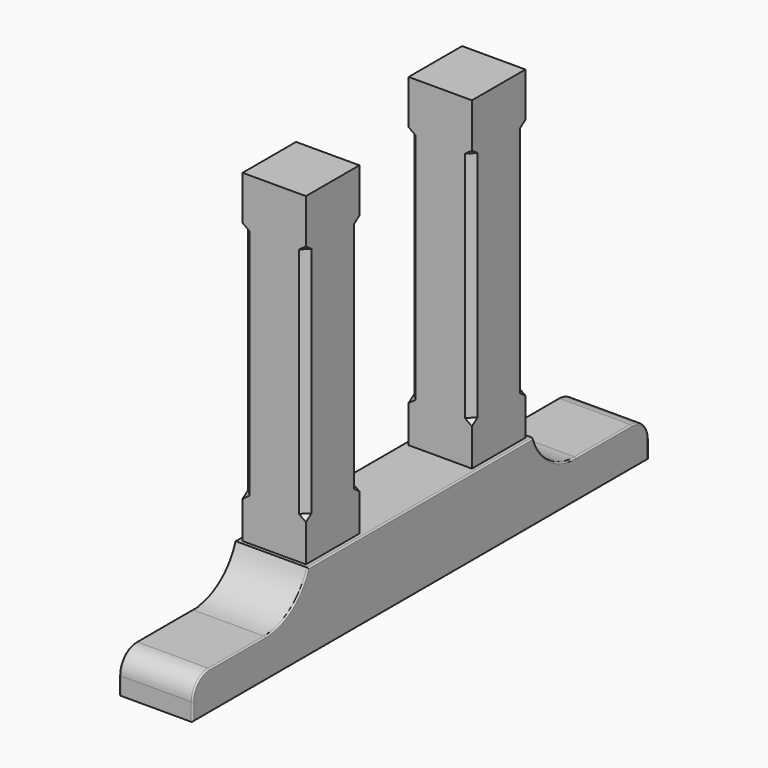
from build123d import *

# Parameters (mm, degrees)
F1_DEPTH      = 52
F1_DEPTH_BACK = 52
F0_W          = 95
F0_H          = 460.873763546
F2_DEPTH      = 45
F2_DEPTH_BACK = 45
F3_R          = 30
F4_T1_DEPTH   = 104
F5_T1_DEPTH   = 104
F6_SIZE       = 10
F7_W          = 90
F7_H          = 95
F8_DEPTH      = 50
F9_W          = 90
F9_H          = 95
F10_DEPTH     = 60
F11_T4_DEPTH  = 65.575795383
F11_T10_DEPTH = 65.575795383
F11_T16_DEPTH = 65.575795383
F11_T22_DEPTH = 65.575795383
F11_T28_DEPTH = 65.575795383
F11_T34_DEPTH = 65.575795383
F11_T40_DEPTH = 65.575795383
F11_T46_DEPTH = 65.575795383
F12_T4_DEPTH  = 65.575795383
F12_T10_DEPTH = 65.575795383
F12_T16_DEPTH = 65.575795383
F12_T22_DEPTH = 65.575795383
F12_T28_DEPTH = 65.575795383
F12_T34_DEPTH = 65.575795383
F12_T40_DEPTH = 65.575795383
F12_T46_DEPTH = 65.575795383
F13_R         = 2


# Not quite as in the source:
# - a fillet or chamfer that OpenCascade refuses, or shapes differently, is made with other operations: its cross-section is extruded or revolved along the edge and cut away or added


with BuildPart() as f1:
    # F0 (on Right) → F1 (new body, two sides)
    with BuildSketch(Plane.YZ) as f1_sk:
        Polygon((-405, 55), (-405, 0), (405, 0), (405, 55), (200, 55), (200, 110), (195, 110), (100, 110), (0, 110), (-100, 110), (-195, 110), (-200, 110), (-200, 55), align=None)
    extrude(amount=F1_DEPTH)
    extrude(f1_sk.sketch, amount=-F1_DEPTH_BACK)

    # F0 (on Right) → F2 (join, two sides)
    with BuildSketch(Plane.YZ) as f2_sk:
        with Locations((-147.5, 340.436881773)):
            Rectangle(F0_W, F0_H)
        with Locations((147.5, 340.436881773)):
            Rectangle(F0_W, F0_H)
    extrude(amount=-F2_DEPTH)
    extrude(f2_sk.sketch, amount=F2_DEPTH_BACK)

    # F3
    f3_edges = [f1.edges().sort_by_distance(p)[0] for p in [
        (0, 405, 55),
        (0, -405, 55),
    ]]
    fillet(f3_edges, radius=F3_R)

    # F4: fillet of radius 80 on 1 edges, made by hand

    # F4_s2 → F4_t1 (join)
    with BuildSketch(Plane.YZ.offset(-52)):
        with BuildLine():
            ThreePointArc((275.9934207679, 55), (229.0892631696, 70.1925930159), (200, 110))
            Line((200, 110), (200, 55))
            Line((200, 55), (275.9934207679, 55))
        make_face()
    extrude(amount=F4_T1_DEPTH)

    # F5: fillet of radius 80 on 1 edges, made by hand

    # F5_s2 → F5_t1 (join)
    with BuildSketch(Plane.YZ.offset(-52)):
        with BuildLine():
            ThreePointArc((-275.9934207679, 55), (-229.0892631696, 70.1925930159), (-200, 110))
            Line((-200, 110), (-200, 55))
            Line((-200, 55), (-275.9934207679, 55))
        make_face()
    extrude(amount=F5_T1_DEPTH)

    # F6
    f6_edges = [f1.edges().sort_by_distance(p)[0] for p in [
        (45, -195, 340.436882),
        (45, -100, 340.436882),
        (45, 100, 340.436882),
        (-45, -195, 340.436882),
        (-45, -100, 340.436882),
        (-45, 100, 340.436882),
        (-45, 195, 340.436882),
        (45, 195, 340.436882),
    ]]
    chamfer(f6_edges, length=F6_SIZE)

    # F7 (on face) → F8 (join)
    with BuildSketch(Plane.XY.offset(110)):
        with Locations((0, -147.5)):
            Rectangle(F7_W, F7_H)
        with Locations((0, 147.5)):
            Rectangle(F7_W, F7_H)
    extrude(amount=F8_DEPTH)

    # F9 (on face) → F10 (join)
    with BuildSketch(Plane.XY.offset(570.873763546)):
        Polygon((45, -110), (45, -100), (35, -100), align=None)
        Polygon((-45, -110), (-35, -100), (-45, -100), align=None)
        Polygon((45, -195), (45, -185), (35, -195), align=None)
        Polygon((-35, -195), (-45, -185), (-45, -195), align=None)
        with Locations((0, 147.5)):
            Rectangle(F9_W, F9_H)
        Polygon((45, -110), (35, -100), (-35, -100), (-45, -110), (-45, -185), (-35, -195), (35, -195), (45, -185), align=None)
    extrude(amount=-F10_DEPTH)

    # F11: chamfer of 10 on 8 edges, made by hand


with BuildPart() as f11_tool2:
    # F11_s3 → F11_t4 (new body)
    with BuildSketch(Plane(origin=(-98.1845447985, -98.1845447985, 0), x_dir=(0, 0, 1), z_dir=(0.7071067812, 0.7071067812, 0))):
        Polygon((510.873763546, 172.6345596729), (500.873763546, 162.6345596729), (510.873763546, 162.6345596729), align=None)
    extrude(amount=F11_T4_DEPTH)

    split(bisect_by=Plane.YZ.offset(45), keep=Keep.BOTTOM)

    split(bisect_by=Plane.XZ.offset(195), keep=Keep.BOTTOM)


with BuildPart() as f1_1:
    add(f1.part)

    # F11_t1: union F11_tool2
    add(f11_tool2.part)


with BuildPart() as f11_tool8:
    # F11_s9 → F11_t10 (new body)
    with BuildSketch(Plane(origin=(49.3154552015, -49.3154552015, 0), x_dir=(0, 0, 1), z_dir=(0.7071067812, -0.7071067812, 0))):
        Polygon((500.873763546, 45.9619407771), (510.873763546, 35.9619407771), (510.873763546, 45.9619407771), align=None)
    extrude(amount=F11_T10_DEPTH)

    split(bisect_by=Plane.YZ.offset(45), keep=Keep.BOTTOM)

    split(bisect_by=Plane.XZ.offset(100), keep=Keep.TOP)


with BuildPart() as f1_2:
    add(f1_1.part)

    # F11_t7: union F11_tool8
    add(f11_tool8.part)


with BuildPart() as f11_tool14:
    # F11_s15 → F11_t16 (new body)
    with BuildSketch(Plane(origin=(-95.6845447985, -95.6845447985, 0), x_dir=(0, 0, 1), z_dir=(0.7071067812, 0.7071067812, 0))):
        Polygon((510.873763546, 35.9619407771), (500.873763546, 45.9619407771), (510.873763546, 45.9619407771), align=None)
    extrude(amount=F11_T16_DEPTH)

    split(bisect_by=Plane.YZ.offset(-45), keep=Keep.TOP)

    split(bisect_by=Plane.XZ.offset(100), keep=Keep.TOP)


with BuildPart() as f1_3:
    add(f1_2.part)

    # F11_t13: union F11_tool14
    add(f11_tool14.part)


with BuildPart() as f11_tool20:
    # F11_s21 → F11_t22 (new body)
    with BuildSketch(Plane(origin=(98.1845447985, -98.1845447985, 0), x_dir=(0, 0, 1), z_dir=(-0.7071067812, 0.7071067812, 0))):
        Polygon((510.873763546, -172.6345596729), (500.873763546, -162.6345596729), (510.873763546, -162.6345596729), align=None)
    extrude(amount=F11_T22_DEPTH)

    split(bisect_by=Plane.XZ.offset(195), keep=Keep.BOTTOM)

    split(bisect_by=Plane.YZ.offset(-45), keep=Keep.TOP)


with BuildPart() as f1_4:
    add(f1_3.part)

    # F11_t19: union F11_tool20
    add(f11_tool20.part)


with BuildPart() as f11_tool26:
    # F11_s27 → F11_t28 (new body)
    with BuildSketch(Plane(origin=(-98.1845447985, 98.1845447985, 0), x_dir=(0, 0, 1), z_dir=(0.7071067812, -0.7071067812, 0))):
        Polygon((500.873763546, -162.6345596729), (510.873763546, -172.6345596729), (510.873763546, -162.6345596729), align=None)
    extrude(amount=F11_T28_DEPTH)

    split(bisect_by=Plane.YZ.offset(45), keep=Keep.BOTTOM)

    split(bisect_by=Plane.XZ.offset(-195), keep=Keep.TOP)


with BuildPart() as f1_5:
    add(f1_4.part)

    # F11_t25: union F11_tool26
    add(f11_tool26.part)


with BuildPart() as f11_tool32:
    # F11_s33 → F11_t34 (new body)
    with BuildSketch(Plane(origin=(49.3154552015, 49.3154552015, 0), x_dir=(0, 0, 1), z_dir=(0.7071067812, 0.7071067812, 0))):
        Polygon((510.873763546, -35.9619407771), (500.873763546, -45.9619407771), (510.873763546, -45.9619407771), align=None)
    extrude(amount=F11_T34_DEPTH)

    split(bisect_by=Plane.YZ.offset(45), keep=Keep.BOTTOM)

    split(bisect_by=Plane.XZ.offset(-100), keep=Keep.BOTTOM)


with BuildPart() as f1_6:
    add(f1_5.part)

    # F11_t31: union F11_tool32
    add(f11_tool32.part)


with BuildPart() as f11_tool38:
    # F11_s39 → F11_t40 (new body)
    with BuildSketch(Plane(origin=(-49.3154552015, 49.3154552015, 0), x_dir=(0, 0, 1), z_dir=(-0.7071067812, 0.7071067812, 0))):
        Polygon((510.873763546, 35.9619407771), (500.873763546, 45.9619407771), (510.873763546, 45.9619407771), align=None)
    extrude(amount=F11_T40_DEPTH)

    split(bisect_by=Plane.XZ.offset(-100), keep=Keep.BOTTOM)

    split(bisect_by=Plane.YZ.offset(-45), keep=Keep.TOP)


with BuildPart() as f1_7:
    add(f1_6.part)

    # F11_t37: union F11_tool38
    add(f11_tool38.part)


with BuildPart() as f11_tool44:
    # F11_s45 → F11_t46 (new body)
    with BuildSketch(Plane(origin=(51.8154552015, 51.8154552015, 0), x_dir=(0, 0, 1), z_dir=(0.7071067812, 0.7071067812, 0))):
        Polygon((510.873763546, -172.6345596729), (500.873763546, -162.6345596729), (510.873763546, -162.6345596729), align=None)
    extrude(amount=F11_T46_DEPTH)

    split(bisect_by=Plane.YZ.offset(-45), keep=Keep.TOP)

    split(bisect_by=Plane.XZ.offset(-195), keep=Keep.TOP)


with BuildPart() as f1_8:
    add(f1_7.part)

    # F11_t43: union F11_tool44
    add(f11_tool44.part)

    # F12: chamfer of 10 on 8 edges, made by hand


with BuildPart() as f12_tool2:
    # F12_s3 → F12_t4 (new body)
    with BuildSketch(Plane(origin=(51.8154552015, 51.8154552015, 0), x_dir=(0, 0, 1), z_dir=(0.7071067812, 0.7071067812, 0))):
        Polygon((170, -162.6345596729), (160, -172.6345596729), (160, -162.6345596729), align=None)
    extrude(amount=F12_T4_DEPTH)

    split(bisect_by=Plane.YZ.offset(-45), keep=Keep.TOP)

    split(bisect_by=Plane.XZ.offset(-195), keep=Keep.TOP)


with BuildPart() as f1_9:
    add(f1_8.part)

    # F12_t1: union F12_tool2
    add(f12_tool2.part)


with BuildPart() as f12_tool8:
    # F12_s9 → F12_t10 (new body)
    with BuildSketch(Plane(origin=(-98.1845447985, 98.1845447985, 0), x_dir=(0, 0, 1), z_dir=(0.7071067812, -0.7071067812, 0))):
        Polygon((160, -172.6345596729), (170, -162.6345596729), (160, -162.6345596729), align=None)
    extrude(amount=F12_T10_DEPTH)

    split(bisect_by=Plane.YZ.offset(45), keep=Keep.BOTTOM)

    split(bisect_by=Plane.XZ.offset(-195), keep=Keep.TOP)


with BuildPart() as f1_10:
    add(f1_9.part)

    # F12_t7: union F12_tool8
    add(f12_tool8.part)


with BuildPart() as f12_tool14:
    # F12_s15 → F12_t16 (new body)
    with BuildSketch(Plane(origin=(49.3154552015, 49.3154552015, 0), x_dir=(0, 0, 1), z_dir=(0.7071067812, 0.7071067812, 0))):
        Polygon((170, -45.9619407771), (160, -35.9619407771), (160, -45.9619407771), align=None)
    extrude(amount=F12_T16_DEPTH)

    split(bisect_by=Plane.YZ.offset(45), keep=Keep.BOTTOM)

    split(bisect_by=Plane.XZ.offset(-100), keep=Keep.BOTTOM)


with BuildPart() as f1_11:
    add(f1_10.part)

    # F12_t13: union F12_tool14
    add(f12_tool14.part)


with BuildPart() as f12_tool20:
    # F12_s21 → F12_t22 (new body)
    with BuildSketch(Plane(origin=(-98.1845447985, -98.1845447985, 0), x_dir=(0, 0, 1), z_dir=(0.7071067812, 0.7071067812, 0))):
        Polygon((170, 162.6345596729), (160, 172.6345596729), (160, 162.6345596729), align=None)
    extrude(amount=F12_T22_DEPTH)

    split(bisect_by=Plane.YZ.offset(45), keep=Keep.BOTTOM)

    split(bisect_by=Plane.XZ.offset(195), keep=Keep.BOTTOM)


with BuildPart() as f1_12:
    add(f1_11.part)

    # F12_t19: union F12_tool20
    add(f12_tool20.part)


with BuildPart() as f12_tool26:
    # F12_s27 → F12_t28 (new body)
    with BuildSketch(Plane(origin=(49.3154552015, -49.3154552015, 0), x_dir=(0, 0, 1), z_dir=(0.7071067812, -0.7071067812, 0))):
        Polygon((160, 35.9619407771), (170, 45.9619407771), (160, 45.9619407771), align=None)
    extrude(amount=F12_T28_DEPTH)

    split(bisect_by=Plane.YZ.offset(45), keep=Keep.BOTTOM)

    split(bisect_by=Plane.XZ.offset(100), keep=Keep.TOP)


with BuildPart() as f1_13:
    add(f1_12.part)

    # F12_t25: union F12_tool26
    add(f12_tool26.part)


with BuildPart() as f12_tool32:
    # F12_s33 → F12_t34 (new body)
    with BuildSketch(Plane(origin=(-95.6845447985, -95.6845447985, 0), x_dir=(0, 0, 1), z_dir=(0.7071067812, 0.7071067812, 0))):
        Polygon((170, 45.9619407771), (160, 35.9619407771), (160, 45.9619407771), align=None)
    extrude(amount=F12_T34_DEPTH)

    split(bisect_by=Plane.YZ.offset(-45), keep=Keep.TOP)

    split(bisect_by=Plane.XZ.offset(100), keep=Keep.TOP)


with BuildPart() as f1_14:
    add(f1_13.part)

    # F12_t31: union F12_tool32
    add(f12_tool32.part)


with BuildPart() as f12_tool38:
    # F12_s39 → F12_t40 (new body)
    with BuildSketch(Plane(origin=(-49.3154552015, 49.3154552015, 0), x_dir=(0, 0, 1), z_dir=(-0.7071067812, 0.7071067812, 0))):
        Polygon((170, 45.9619407771), (160, 35.9619407771), (160, 45.9619407771), align=None)
    extrude(amount=F12_T40_DEPTH)

    split(bisect_by=Plane.XZ.offset(-100), keep=Keep.BOTTOM)

    split(bisect_by=Plane.YZ.offset(-45), keep=Keep.TOP)


with BuildPart() as f1_15:
    add(f1_14.part)

    # F12_t37: union F12_tool38
    add(f12_tool38.part)


with BuildPart() as f12_tool44:
    # F12_s45 → F12_t46 (new body)
    with BuildSketch(Plane(origin=(98.1845447985, -98.1845447985, 0), x_dir=(0, 0, 1), z_dir=(-0.7071067812, 0.7071067812, 0))):
        Polygon((170, -162.6345596729), (160, -172.6345596729), (160, -162.6345596729), align=None)
    extrude(amount=F12_T46_DEPTH)

    split(bisect_by=Plane.XZ.offset(195), keep=Keep.BOTTOM)

    split(bisect_by=Plane.YZ.offset(-45), keep=Keep.TOP)


with BuildPart() as f1_16:
    add(f1_15.part)

    # F12_t43: union F12_tool44
    add(f12_tool44.part)

    # F13
    f13_edges = [f1_16.edges().sort_by_distance(p)[0] for p in [
        (52, -405, 12.5),
        (52, 0, 0),
        (52, 405, 12.5),
        (52, 396.213203, 46.213203),
        (52, 325.49671, 55),
        (52, 229.089263, 70.192593),
        (52, 0, 110),
        (52, -229.089263, 70.192593),
        (52, -325.49671, 55),
        (52, -396.213203, 46.213203),
        (-52, -405, 12.5),
        (-52, 0, 0),
        (-52, 405, 12.5),
        (-52, 396.213203, 46.213203),
        (-52, 325.49671, 55),
        (-52, 229.089263, 70.192593),
        (-52, 0, 110),
        (-52, -229.089263, 70.192593),
        (-52, -325.49671, 55),
        (-52, -396.213203, 46.213203),
    ]]
    fillet(f13_edges, radius=F13_R)


solid = f1_16.part
